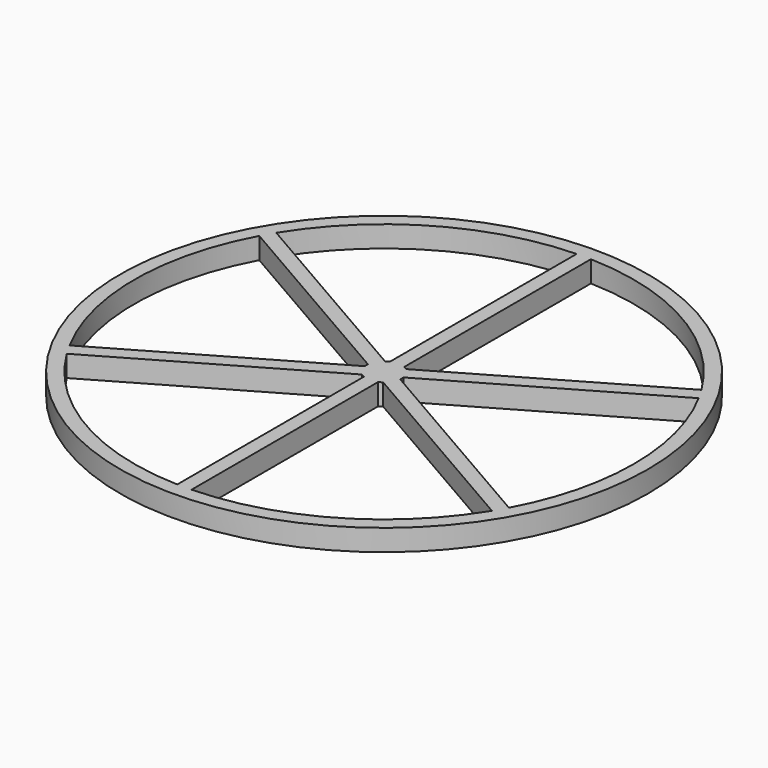
from build123d import *

# Parameters (mm, degrees)
F0_R            = 37
F1_DEPTH        = 3
F2_DEPTH        = 3
F2_COPIES_COUNT = 6


# Not quite as in the source:
# - a pattern or mirror of a feature is missing from the dataset's text; its kind, count and spacing are read off the source's solid


with BuildPart() as f1:
    # F0 (on Top) → F1 (new body)
    with BuildSketch(Plane.XY):
        Circle(F0_R)
        with BuildLine():
            Line((1, 35.6262177595), (1, 34.9857113691))
            ThreePointArc((1, 34.9857113691), (25.099800796, 24.3926218353), (35, 0))
            ThreePointArc((35, 0), (-24.3926218353, -25.099800796), (-1, 34.9857113691))
            Line((-1, 34.9857113691), (-1, 35.6262177595))
            Line((-1, 35.6262177595), (1, 35.6262177595))
        make_face(mode=Mode.SUBTRACT)
        with BuildLine():
            ThreePointArc((-1, 34.9857113691), (0, 35), (1, 34.9857113691))
            Line((1, 34.9857113691), (1, 35.6262177595))
            Line((1, 35.6262177595), (-1, 35.6262177595))
            Line((-1, 35.6262177595), (-1, 34.9857113691))
        make_face()
    extrude(amount=F1_DEPTH)



with BuildPart() as f1b:
    # F0 (on Top) → F1, piece 2 (new body)
    with BuildSketch(Plane.XY):
        with BuildLine():
            ThreePointArc((-1, 2.2912878475), (-1.3693063938, -2.0916500663), (2.5, 0))
            ThreePointArc((2.5, 0), (2.0916500663, 1.3693063938), (1, 2.2912878475))
            Line((1, 2.2912878475), (1, 0.5877822405))
            Line((1, 0.5877822405), (-1, 0.5877822405))
            Line((-1, 0.5877822405), (-1, 2.2912878475))
        make_face()
        with BuildLine():
            Line((1, 0.5877822405), (1, 2.2912878475))
            ThreePointArc((1, 2.2912878475), (0, 2.5), (-1, 2.2912878475))
            Line((-1, 2.2912878475), (-1, 0.5877822405))
            Line((-1, 0.5877822405), (1, 0.5877822405))
        make_face()
    extrude(amount=F1_DEPTH)


with BuildPart() as f1_1:
    add(f1.part)

    add(f1b.part)  # F2 merges F1b
    # F0 (on Top) → F2 (join)
    with BuildSketch(Plane.XY):
        with BuildLine():
            Line((1, 0.5877822405), (1, 2.2912878475))
            ThreePointArc((1, 2.2912878475), (0, 2.5), (-1, 2.2912878475))
            Line((-1, 2.2912878475), (-1, 0.5877822405))
            Line((-1, 0.5877822405), (1, 0.5877822405))
        make_face()
        with BuildLine():
            ThreePointArc((-1, 2.2912878475), (0, 2.5), (1, 2.2912878475))
            Line((1, 2.2912878475), (1, 34.9857113691))
            ThreePointArc((1, 34.9857113691), (0, 35), (-1, 34.9857113691))
            Line((-1, 34.9857113691), (-1, 2.2912878475))
        make_face()
        with BuildLine():
            ThreePointArc((-1, 34.9857113691), (0, 35), (1, 34.9857113691))
            Line((1, 34.9857113691), (1, 35.6262177595))
            Line((1, 35.6262177595), (-1, 35.6262177595))
            Line((-1, 35.6262177595), (-1, 34.9857113691))
        make_face()
    f2 = extrude(amount=F2_DEPTH)

    # F2_copies: F2 ×6 about axis
    f2_copies_axis = Axis((0, 0, 0), (0, 0, 1))
    for i in range(1, F2_COPIES_COUNT):
        add(f2.rotate(f2_copies_axis, i * 360 / F2_COPIES_COUNT))


solid = f1_1.part
